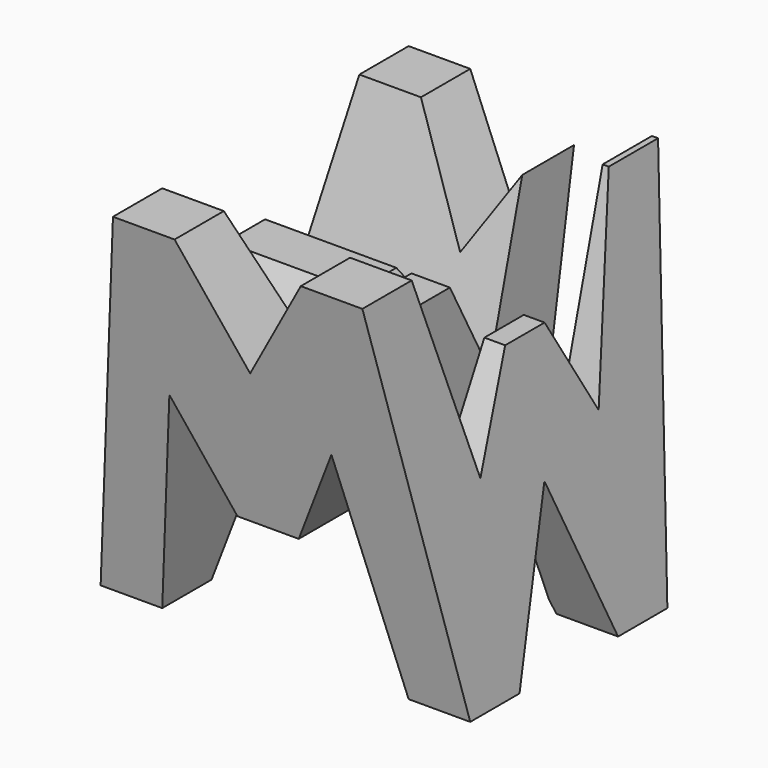
from build123d import *

# Parameters (mm, degrees)
F0_W     = 38.1
F0_H     = 38.1
F1_DEPTH = 38.1
F5_DEPTH = 38.1
F7_DEPTH = 38.1
F9_DEPTH = 38.1


with BuildPart() as f1:
    # F0 (on Front) → F1 (new body)
    with BuildSketch(Plane.XZ):
        with Locations((47.4635573444, 19.05)):
            Rectangle(F0_W, F0_H)
    extrude(amount=F1_DEPTH)

    # F4 (on face) → F5 (cut)
    with BuildSketch(Plane.YZ.offset(66.5135573444)):
        Polygon((-31.75, 0), (-38.1, 38.1), (-38.1, 0), align=None)
        Polygon((-6.35, 38.1), (-31.75, 38.1), (-26.67, 19.0584023679), (-21.59, 28.575), (-16.51, 28.575), (-11.43, 19.0584023679), align=None)
        Polygon((0, 0), (0, 38.1), (-6.35, 0), align=None)
        Polygon((-19.05, 15.875), (-25.4, 0), (-12.7, 0), align=None)
    extrude(amount=-F5_DEPTH, mode=Mode.SUBTRACT)

    # F6 (on offset) → F7 (cut)
    with BuildSketch(Plane.XZ.offset(38.1)):
        Polygon((38.4384175691, 22.0491613483), (34.7635573444, 0), (60.1635573444, 0), (55.1432829689, 22.0491613483), (50.4643332552, 12.2184510259), (44.1477571021, 12.2184510259), align=None)
        Polygon((34.7635573444, 38.1), (28.4135573444, 38.1), (28.4135573444, 0), align=None)
        Polygon((54.1253941298, 38.1), (41.1135573444, 38.1), (47.4635573444, 27.2768866271), align=None)
        Polygon((60.4753941298, 38.1), (66.5135573444, 0), (66.5135573444, 38.1), align=None)
    extrude(amount=-F7_DEPTH, mode=Mode.SUBTRACT)

    # F8 (on offset) → F9 (cut)
    with BuildSketch(Plane.XY.offset(38.1)):
        Polygon((59.8412752151, 0), (52.2212752151, 0), (52.2212752151, -12.7), (52.2212752151, -25.3993560767), (59.8412752151, -25.3993560767), (59.8412752151, -12.6993560767), align=None)
    extrude(amount=-F9_DEPTH, mode=Mode.SUBTRACT)


solid = f1.part
